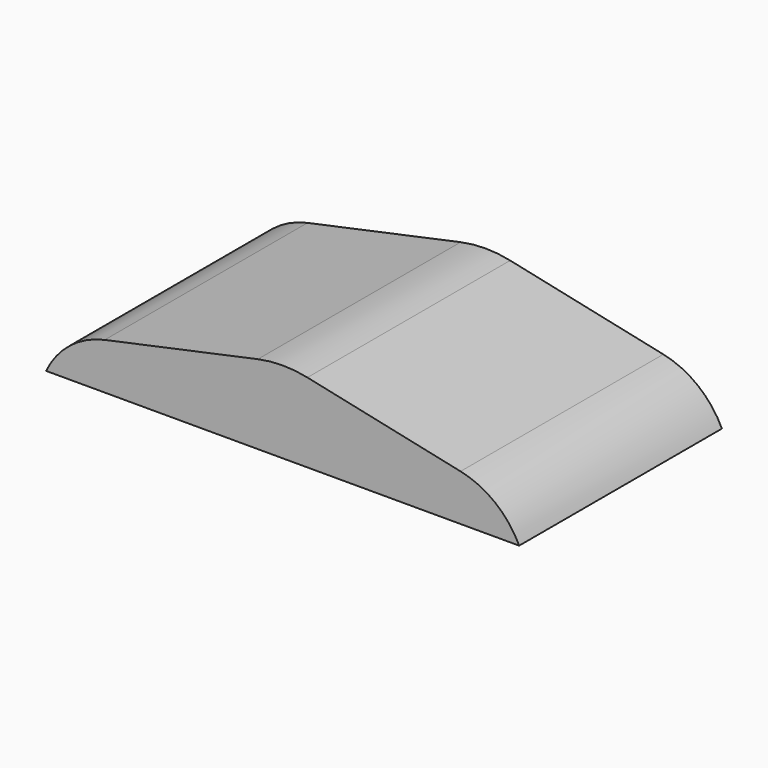
from build123d import *

# Parameters (mm, degrees)
F1_DEPTH    = 15
F2_T1_DEPTH = 32.7362862295
F3_R        = 7


# Not quite as in the source:
# - a fillet or chamfer that OpenCascade refuses, or shapes differently, is made with other operations: its cross-section is extruded or revolved along the edge and cut away or added


with BuildPart() as f1:
    # F0 (on Front) → F1 (new body)
    with BuildSketch(Plane.XZ):
        Polygon((-14, 0), (14, 0), (14, 2), (0, 5), (-14, 2), align=None)
    extrude(amount=F1_DEPTH)

    # F2: fillet of radius 5 on 2 edges, made by hand

    # F2_s2 → F2_t1 (cut)
    with BuildSketch(Plane.XZ.offset(-8.8681431148)):
        with BuildLine():
            ThreePointArc((-10.5314833016, 2.7432535782), (-12.5855065639, 1.7759313526), (-14, 0))
            Line((-14, 0), (-14, 2))
            Line((-14, 2), (-10.5314833016, 2.7432535782))
        make_face()
        with BuildLine():
            ThreePointArc((14, 0), (12.5855065639, 1.7759313526), (10.5314833016, 2.7432535782))
            Line((10.5314833016, 2.7432535782), (14, 2))
            Line((14, 2), (14, 0))
        make_face()
    extrude(amount=F2_T1_DEPTH, mode=Mode.SUBTRACT)

    # F3
    f3_edges = [f1.edges().sort_by_distance(p)[0] for p in [
        (0, -7.5, 5),
    ]]
    fillet(f3_edges, radius=F3_R)


solid = f1.part
